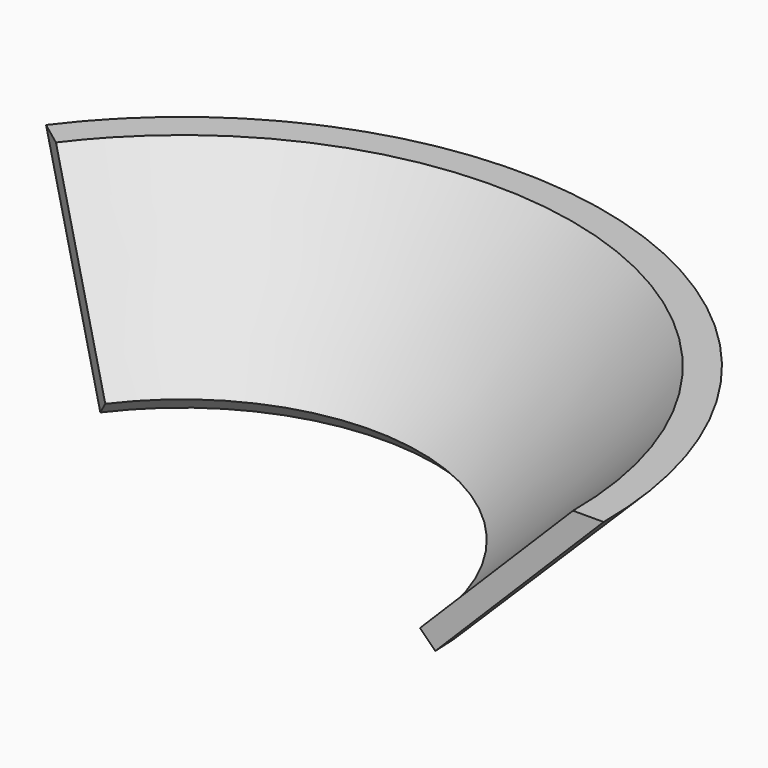
from build123d import *

# Parameters (mm, degrees)
F1_ANGLE = 143.2394
F2_SIZE2 = 1.999
F2_SIZE  = 1.999


# Not quite as in the source:
# - a fillet or chamfer is up to 0.001 mm smaller than in the source, because OpenCascade refuses the exact size
# - a feature names something its author has since deleted; it is built from what else it names


with BuildPart() as f1:
    # F0 (on Front) → F1 (revolve)
    with BuildSketch(Plane.XZ):
        Polygon((23.4142135624, 0), (38.9705627485, 15.5563491861), (37.5563491861, 16.9705627485), (22, 1.4142135624), align=None)
    revolve(axis=Axis((0, 0, 11), (0, 0, 1)), revolution_arc=F1_ANGLE)

    # F2 (size 2 and 2 in the source; OpenCascade refuses exactly that, so slightly less here)
    f2_edges = [f1.edges().sort_by_distance(p)[0] for p in [
        (11.842372, 35.640393, 16.970563),
    ]]
    chamfer(f2_edges, length=F2_SIZE, length2=F2_SIZE2)


solid = f1.part
